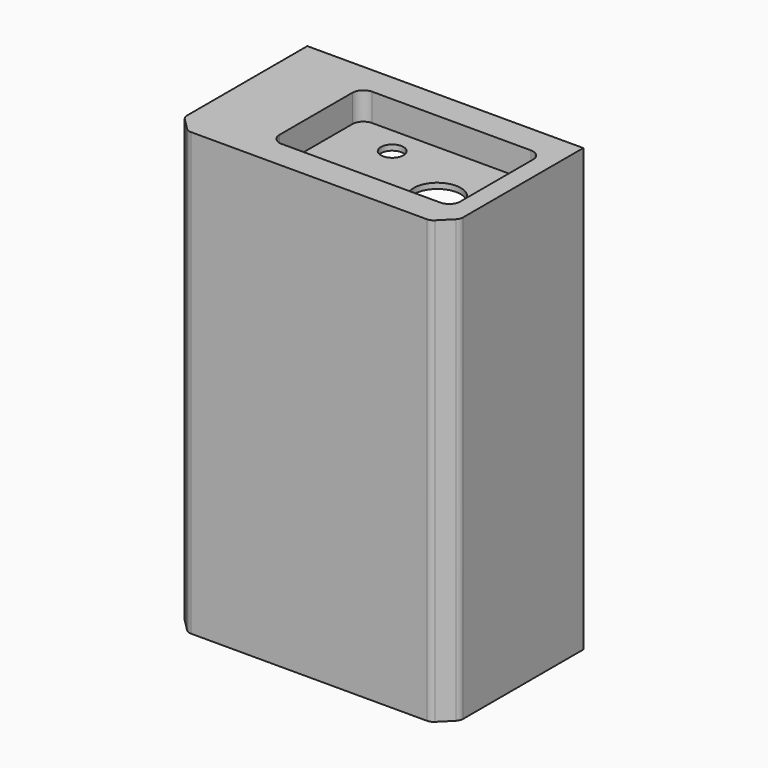
from build123d import *

# Parameters (mm, degrees)
F1_W      = 50
F1_H      = 27.68
F1_W_2    = 47.8036555797
F1_H_2    = 25.68
F2_DEPTH  = 80
F1_W_3    = 34.129309468
F1_H_3    = 21.4303236678
F1_W_4    = 32.75
F1_H_4    = 20.5
F3_DEPTH  = 6
F0_W      = 32.75
F0_H      = 20.5
F0_R      = 2.05
F0_R_2    = 4.25
F4_DEPTH  = 6
F5_DEPTH  = 5
F6_DEPTH  = 1
F7_R      = 2
F8_W      = 50
F8_H      = 80
F9_DEPTH  = 1
F10_ANGLE = 180
F11_W     = 47.8036555797
F11_H     = 25.68
F12_DEPTH = 1
F13_W     = 8
F13_H     = 8
F14_DEPTH = 8
F15_W     = 8
F15_H     = 8
F16_DEPTH = 8
F19_SIZE  = 2
F20_SIZE  = 3
F21_R     = 1.5
F22_R     = 1
F18_R     = 2.55
F23_DEPTH = 5.1
F24_W     = 50
F24_H     = 80
F25_DEPTH = 4.18


with BuildPart() as f2:
    # F1 (on face) → F2 (new body)
    with BuildSketch(Plane.XY):
        Rectangle(F1_W, F1_H)
        with Locations((-0.0981722102, 0)):
            Rectangle(F1_W_2, F1_H_2, mode=Mode.SUBTRACT)
    extrude(amount=F2_DEPTH)

    # F8 (on face) → F9 (cut)
    with BuildSketch(Plane.XZ.offset(13.84)):
        with Locations((0, 40)):
            Rectangle(F8_W, F8_H)
    extrude(amount=-F9_DEPTH, mode=Mode.SUBTRACT)


with BuildPart() as f3:
    # F1 (on face) → F3 (new body)
    with BuildSketch(Plane.XY):
        with Locations((5.3276410885, -1.4191564249)):
            Rectangle(F1_W_3, F1_H_3)
        with Locations((5.28, -1.59)):
            Rectangle(F1_W_4, F1_H_4, mode=Mode.SUBTRACT)
    extrude(amount=F3_DEPTH)

    # F0 (on Top) → F4 (join)
    with BuildSketch(Plane.XY):
        with Locations((5.28, -1.59)):
            Rectangle(F0_W, F0_H)
        with Locations((-1.515, -6.89)):
            Circle(F0_R, mode=Mode.SUBTRACT)
        with Locations((12.16, 0)):
            Circle(F0_R_2, mode=Mode.SUBTRACT)
    extrude(amount=F4_DEPTH)

    # F1 (on face) → F5 (cut)
    with BuildSketch(Plane.XY):
        with Locations((5.28, -1.59)):
            Rectangle(F1_W_4, F1_H_4)
    extrude(amount=F5_DEPTH, mode=Mode.SUBTRACT)

    # F7
    f7_edges = [f3.edges().sort_by_distance(p)[0] for p in [
        (21.655, -11.84, 2.5),
        (-11.095, -11.84, 2.5),
        (21.655, 8.66, 2.5),
        (-11.095, 8.66, 2.5),
    ]]
    fillet(f7_edges, radius=F7_R)


with BuildPart() as f6:
    # F1 (on face) → F6 (new body)
    with BuildSketch(Plane.XY):
        with Locations((-0.0981722102, 0)):
            Rectangle(F1_W_2, F1_H_2)
        with Locations((5.3276410885, -1.4191564249)):
            Rectangle(F1_W_3, F1_H_3, mode=Mode.SUBTRACT)
    extrude(amount=F6_DEPTH)


with BuildPart() as f6_1:
    # F10: moved
    add(f6.part.rotate(Axis((-0.0981722102, -12.84, 0), (1, 0, 0)), F10_ANGLE))


with BuildPart() as f2_1:
    # F10: moved
    add(f2.part.rotate(Axis((-0.0981722102, -12.84, 0), (1, 0, 0)), F10_ANGLE))

    # F11 (on face) → F12 (join)
    with BuildSketch(Plane(origin=(0, 0, -80), x_dir=(1, 0, 0), z_dir=(0, 0, -1))):
        with Locations((-0.0981722102, 25.68)):
            Rectangle(F11_W, F11_H)
    extrude(amount=-F12_DEPTH)


    add(f6_1.part)  # F14 merges F6
    # F13 (on face) → F14 (join)
    with BuildSketch(Plane.YZ.offset(-24)):
        with Locations((-16.84, -5)):
            Rectangle(F13_W, F13_H)
    extrude(amount=F14_DEPTH)

    # F15 (on face) → F16 (join)
    with BuildSketch(Plane(origin=(23.8036555797, 0, 0), x_dir=(0, -1, 0), z_dir=(-1, 0, 0))):
        with Locations((16.84, -75)):
            Rectangle(F15_W, F15_H)
    extrude(amount=F16_DEPTH)


with BuildPart() as f3_1:
    # F10: moved
    add(f3.part.rotate(Axis((-0.0981722102, -12.84, 0), (1, 0, 0)), F10_ANGLE))


with BuildPart() as f2_2:
    add(f2_1.part)

    # F17: union F3
    add(f3_1.part)

    # F19
    f19_edges = [f2_2.edges().sort_by_distance(p)[0] for p in [
        (23.803656, -38.52, -40),
        (-24, -38.52, -40),
    ]]
    chamfer(f19_edges, length=F19_SIZE)

    # F20
    f20_edges = [f2_2.edges().sort_by_distance(p)[0] for p in [
        (-25, -39.52, -40),
        (25, -39.52, -40),
    ]]
    chamfer(f20_edges, length=F20_SIZE)

    # F21
    f21_edges = [f2_2.edges().sort_by_distance(p)[0] for p in [
        (25, -36.52, -40),
        (22, -39.52, -40),
        (-22, -39.52, -40),
        (-25, -36.52, -40),
    ]]
    fillet(f21_edges, radius=F21_R)

    # F22
    f22_edges = [f2_2.edges().sort_by_distance(p)[0] for p in [
        (-24, -16.84, -9),
        (-20, -20.84, -9),
        (-16, -16.84, -9),
        (-16, -20.84, -5),
        (-16, -16.84, -1),
        (15.803656, -16.84, -71),
        (23.803656, -16.84, -71),
        (15.803656, -16.84, -79),
        (15.803656, -20.84, -75),
        (19.803656, -20.84, -71),
        (-11.737014, -24.260844, -1),
        (22.392296, -24.260844, -1),
        (-20, -20.84, -1),
        (23.803656, -20.84, -75),
        (19.803656, -20.84, -79),
        (-24, -20.84, -5),
    ]]
    fillet(f22_edges, radius=F22_R)

    # F18 (on face) → F23 (cut)
    with BuildSketch(Plane(origin=(0, -12.84, 0), x_dir=(-1, 0, 0), z_dir=(0, 1, 0))):
        with Locations((20, -5)):
            Circle(F18_R)
        with Locations((-19.8036555797, -75)):
            Circle(F18_R)
    extrude(amount=-F23_DEPTH, mode=Mode.SUBTRACT)

    # F24 (on face) → F25 (join)
    with BuildSketch(Plane(origin=(0, -12.84, 0), x_dir=(-1, 0, 0), z_dir=(0, 1, 0))):
        with Locations((0, -40)):
            Rectangle(F24_W, F24_H)
        Polygon((-23.8036555797, -70), (-23.8036555797, -1), (15, -1), (24, -1), (24, -10), (24, -79), (-14.8036555797, -79), (-23.8036555797, -79), align=None, mode=Mode.SUBTRACT)
    extrude(amount=F25_DEPTH)


solid = f2_2.part
